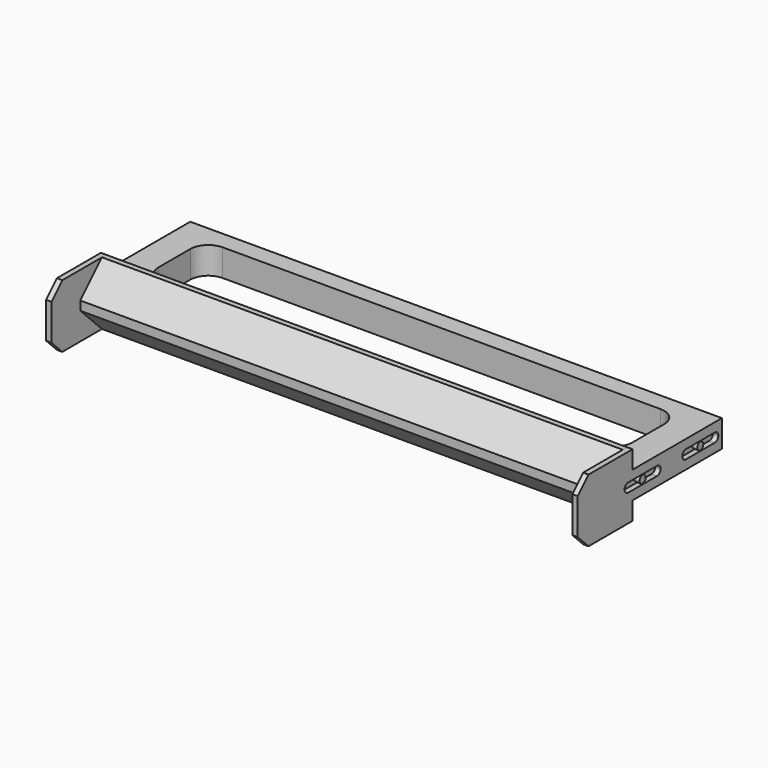
from build123d import *

# Parameters (mm, degrees)
F1_DEPTH       = 17.5
F1_DEPTH_BACK  = 17.5
F2_SIZE        = 15
F3_SIZE        = 7.5
F5_W           = 3
F5_H           = 92.5
F6_DEPTH       = 0.01
F7_W           = 3
F7_H           = 92.5
F8_DEPTH       = 0.01
F4_R           = 2.1
F9_DEPTH       = 3
F11_DEPTH      = 10
F13_DEPTH      = 10
F15_DEPTH      = 25
F16_W          = 295
F16_H          = 62
F17_DEPTH      = 10
F17_DEPTH_BACK = 25
F18_W          = 295
F18_H          = 62
F19_DEPTH      = 10
F19_DEPTH_BACK = 25


with BuildPart() as f1:
    # F0 (on Top) → F1 (new body, two sides)
    with BuildSketch(Plane.XY) as f1_sk:
        Polygon((147.5, -50), (147.5, 50), (-147.5, 50), (-147.5, -50), (-144.5, -50), (-144.5, -30), (144.5, -30), (144.5, -50), align=None)
    extrude(amount=F1_DEPTH)
    extrude(f1_sk.sketch, amount=-F1_DEPTH_BACK)

    # F2
    f2_edges = [f1.edges().sort_by_distance(p)[0] for p in [
        (0, -30, 17.5),
        (0, -30, -17.5),
    ]]
    chamfer(f2_edges, length=F2_SIZE)

    # F3
    f3_edges = [f1.edges().sort_by_distance(p)[0] for p in [
        (146, -50, 17.5),
        (146, -50, -17.5),
        (-146, -50, 17.5),
        (-146, -50, -17.5),
    ]]
    chamfer(f3_edges, length=F3_SIZE)

    # F5 (on face) → F6 (join)
    with BuildSketch(Plane.XY.offset(17.5)):
        with Locations((-146, 3.75)):
            Rectangle(F5_W, F5_H)
        with Locations((146, 3.75)):
            Rectangle(F5_W, F5_H)
    extrude(amount=F6_DEPTH)

    # F7 (on face) → F8 (join)
    with BuildSketch(Plane(origin=(0, 0, -17.5), x_dir=(1, 0, 0), z_dir=(0, 0, -1))):
        with Locations((-146, -3.75)):
            Rectangle(F7_W, F7_H)
        with Locations((146, -3.75)):
            Rectangle(F7_W, F7_H)
    extrude(amount=F8_DEPTH)

    # F4 (on face) → F9 (cut)
    with BuildSketch(Plane.YZ.offset(147.5)):
        with BuildLine():
            ThreePointArc((47.5, 0), (46.767766953, 1.767766953), (45, 2.5))
            Line((45, 2.5), (25, 2.5))
            ThreePointArc((25, 2.5), (23.232233047, 1.767766953), (22.5, 0))
            ThreePointArc((22.5, 0), (23.232233047, -1.767766953), (25, -2.5))
            Line((25, -2.5), (45, -2.5))
            ThreePointArc((45, -2.5), (46.767766953, -1.767766953), (47.5, 0))
        make_face()
        with Locations((35, 0)):
            Circle(F4_R, mode=Mode.SUBTRACT)
        with BuildLine():
            ThreePointArc((7.5, 0), (6.767766953, 1.767766953), (5, 2.5))
            Line((5, 2.5), (-15, 2.5))
            ThreePointArc((-15, 2.5), (-16.767766953, 1.767766953), (-17.5, 0))
            ThreePointArc((-17.5, 0), (-16.767766953, -1.767766953), (-15, -2.5))
            Line((-15, -2.5), (5, -2.5))
            ThreePointArc((5, -2.5), (6.767766953, -1.767766953), (7.5, 0))
        make_face()
        with Locations((-5, 0)):
            Circle(F4_R, mode=Mode.SUBTRACT)
    extrude(amount=-F9_DEPTH, mode=Mode.SUBTRACT)

    # F10 (on face) → F11 (cut)
    with BuildSketch(Plane.XY.offset(17.5)):
        with BuildLine():
            Line((141.5, 50), (-141.5, 50))
            Line((-141.5, 50), (-141.5, -2))
            ThreePointArc((-141.5, -2), (-138.5710678119, -9.0710678119), (-131.5, -12))
            Line((-131.5, -12), (131.5, -12))
            ThreePointArc((131.5, -12), (138.5710678119, -9.0710678119), (141.5, -2))
            Line((141.5, -2), (141.5, 50))
        make_face()
    extrude(amount=-F11_DEPTH, mode=Mode.SUBTRACT)

    # F12 (on face) → F13 (cut)
    with BuildSketch(Plane(origin=(0, 0, -17.5), x_dir=(1, 0, 0), z_dir=(0, 0, -1))):
        with BuildLine():
            Line((141.5, -50), (141.5, 2))
            ThreePointArc((141.5, 2), (138.5710678119, 9.0710678119), (131.5, 12))
            Line((131.5, 12), (-131.5, 12))
            ThreePointArc((-131.5, 12), (-138.5710678119, 9.0710678119), (-141.5, 2))
            Line((-141.5, 2), (-141.5, -50))
            Line((-141.5, -50), (141.5, -50))
        make_face()
    extrude(amount=-F13_DEPTH, mode=Mode.SUBTRACT)

    # F14 (on face) → F15 (cut)
    with BuildSketch(Plane.XY.offset(7.5)):
        with BuildLine():
            Line((121.5, 40), (-121.5, 40))
            ThreePointArc((-121.5, 40), (-128.5710678119, 37.0710678119), (-131.5, 30))
            Line((-131.5, 30), (-131.5, 8))
            ThreePointArc((-131.5, 8), (-128.5710678119, 0.9289321881), (-121.5, -2))
            Line((-121.5, -2), (121.5, -2))
            ThreePointArc((121.5, -2), (128.5710678119, 0.9289321881), (131.5, 8))
            Line((131.5, 8), (131.5, 30))
            ThreePointArc((131.5, 30), (128.5710678119, 37.0710678119), (121.5, 40))
        make_face()
    extrude(amount=-F15_DEPTH, mode=Mode.SUBTRACT)

    # F16 (on face) → F17 (cut, two sides)
    with BuildSketch(Plane.XY.offset(17.5)) as f17_sk:
        with Locations((0, 19)):
            Rectangle(F16_W, F16_H)
    extrude(amount=-F17_DEPTH, mode=Mode.SUBTRACT)
    extrude(f17_sk.sketch, amount=F17_DEPTH_BACK, mode=Mode.SUBTRACT)

    # F18 (on face) → F19 (cut, two sides)
    with BuildSketch(Plane(origin=(0, 0, -17.5), x_dir=(1, 0, 0), z_dir=(0, 0, -1))) as f19_sk:
        with Locations((0, -19)):
            Rectangle(F18_W, F18_H)
    extrude(amount=-F19_DEPTH, mode=Mode.SUBTRACT)
    extrude(f19_sk.sketch, amount=F19_DEPTH_BACK, mode=Mode.SUBTRACT)


solid = f1.part
